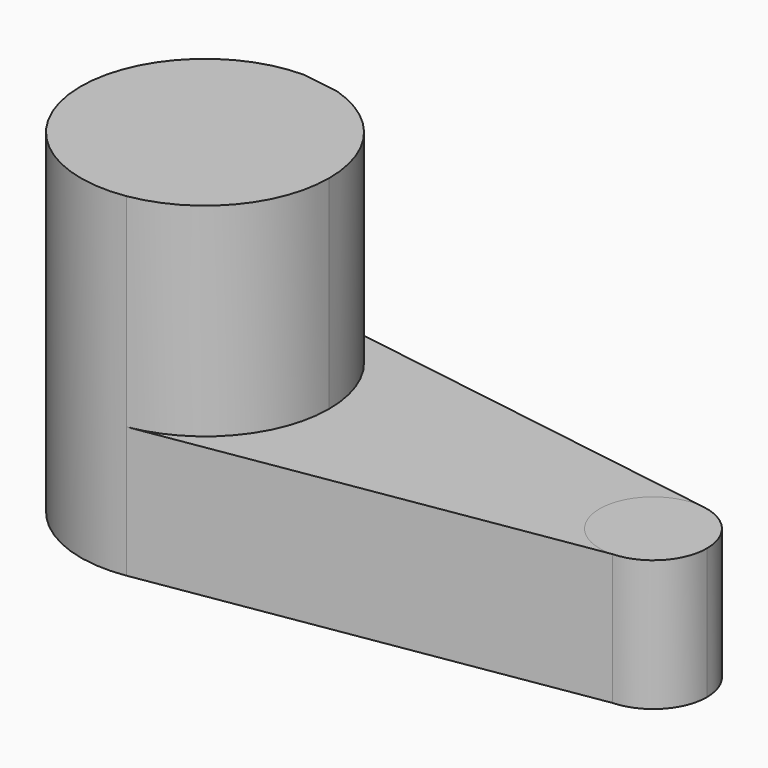
from build123d import *

# Parameters (mm, degrees)
F3_DEPTH = 15.7734
F4_DEPTH = 40.2336


with BuildPart() as f3:
    # F1 (on face) → F3 (new body)
    with BuildSketch(Plane.XY):
        with BuildLine():
            Line((2.3665023004, -14.7686997904), (54.2445329823, -6.4558851165))
            ThreePointArc((54.2445329823, -6.4558851165), (47.5237977676, 0.3648156016), (54.9706478921, 6.3843391154))
            Line((54.9706478921, 6.3843391154), (4.5544000586, 14.246833569))
            ThreePointArc((4.5544000586, 14.246833569), (12.0796407574, 8.8202667652), (14.9570995396, 0))
            ThreePointArc((14.9570995396, 0), (11.3822413677, -9.7035770768), (2.3665023004, -14.7686997904))
        make_face()
    extrude(amount=F3_DEPTH)

    # F0 (on Top) → F4 (join)
    with BuildSketch(Plane.XY):
        with BuildLine():
            ThreePointArc((14.9570995396, 0), (12.0796407574, 8.8202667652), (4.5544000586, 14.246833569))
            Line((4.5544000586, 14.246833569), (0, 14.9570995396))
            ThreePointArc((0, 14.9570995396), (-14.9099252089, -1.1869949034), (2.3665023004, -14.7686997904))
            ThreePointArc((2.3665023004, -14.7686997904), (11.3822413677, -9.7035770768), (14.9570995396, 0))
        make_face()
    extrude(amount=F4_DEPTH)


with BuildPart() as f3b:
    # F2 (on face) → F3, piece 2 (new body)
    with BuildSketch(Plane.XY):
        with BuildLine():
            ThreePointArc((54.9706478921, 6.3843391154), (47.5237977676, 0.3648156016), (54.2445329823, -6.4558851165))
            ThreePointArc((54.2445329823, -6.4558851165), (58.6382976798, -4.472667595), (60.4365091632, 0))
            ThreePointArc((60.4365091632, 0), (58.8833851033, 4.2022442033), (54.9706478921, 6.3843391154))
        make_face()
    extrude(amount=F3_DEPTH)


solid = Compound([f3.part, f3b.part])
